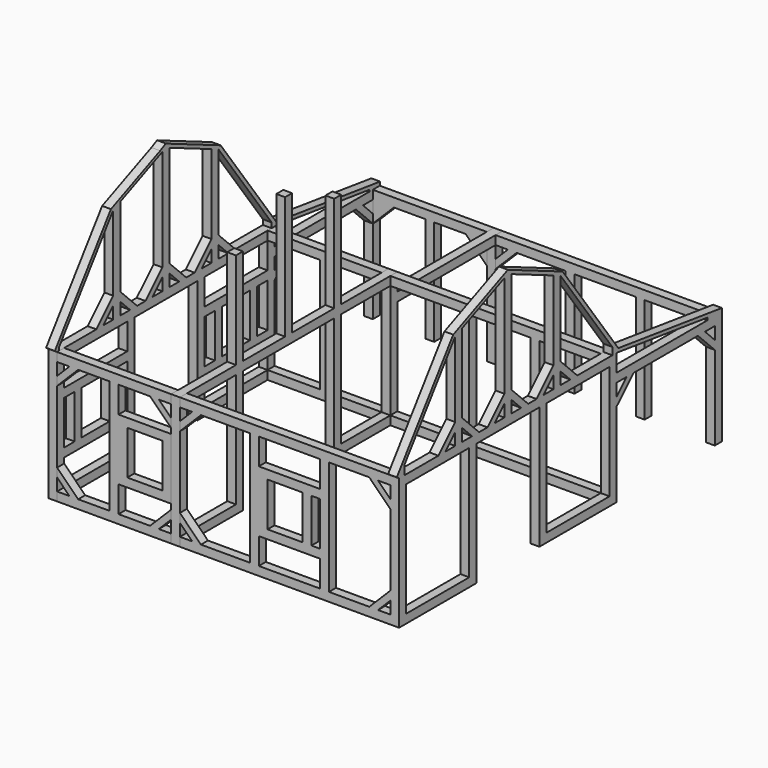
from build123d import *

# Parameters (mm, degrees)
F0_W      = 20
F0_H      = 25
F1_DEPTH  = 5
F0_W_2    = 35
F0_H_2    = 15
F0_W_3    = 5
F2_W      = 7.5
F2_H      = 25
F2_W_2    = 45
F2_H_2    = 15
F2_H_3    = 24.9999969228
F2_W_3    = 20
F3_DEPTH  = 5
F4_W      = 45
F4_H      = 65
F5_DEPTH  = 5
F6_W      = 35
F6_H      = 65
F7_DEPTH  = 5
F8_W      = 35
F8_H      = 65
F9_DEPTH  = 5
F11_DEPTH = 5


# Not quite as in the source:
# - ends of sketch curves that miss each other by under 0.0002 mm in the source are joined


with BuildPart() as f1:
    # F0 (on Front) → F1 (new body)
    with BuildSketch(Plane.XZ):
        Polygon((-8.9761292934, 70), (-73.9761292934, 70), (-73.9761292934, 65), (-66.9761292934, 65), (-73.9761292934, 58), (-73.9761292934, 53), (-61.9761292934, 65), (-43.9761292934, 65), (-43.9761292934, 0), (-61.9761292934, 0), (-73.9761292934, 12), (-73.9761292934, 7), (-66.9761292934, 0), (-73.9761292934, 0), (-73.9761292934, -5), (-8.9761292934, -5), (-8.9761292934, 0), (-15.9761292934, 0), (-8.9761292934, 7), (-8.9761292934, 12), (-20.9761292934, 0), (-38.9761292934, 0), (-38.9761292934, 15), (-8.9761292934, 15), (-8.9761292934, 50), (-38.9761292934, 50), (-38.9761292934, 65), (-20.9761292934, 65), (-8.9761292934, 53), (-8.9761292934, 58), (-15.9761292934, 65), (-8.9761292934, 65), align=None)
        with Locations((-23.9761292934, 32.5)):
            Rectangle(F0_W, F0_H, mode=Mode.SUBTRACT)
    extrude(amount=F1_DEPTH)


with BuildPart() as f1b:
    # F0 (on Front) → F1, piece 2 (new body)
    with BuildSketch(Plane.XZ):
        Polygon((-3.9761292934, -5), (116.0238707066, -5), (116.0238707066, 0), (109.0238707066, 0), (116.0238707066, 7), (116.0238707066, 12), (104.0238707066, 0), (81.0238707066, 0), (81.0238707066, 65), (104.0238707066, 65), (116.0238707066, 53), (116.0238707066, 58), (109.0238707066, 65), (116.0238707066, 65), (116.0238707066, 70), (-3.9761292934, 70), (-3.9761292934, 65), (3.0238707066, 65), (-3.9761292934, 58), (-3.9761292934, 53), (8.0238707066, 65), (36.0238707066, 65), (36.0238707066, 0), (8.0238707066, 0), (-3.9761292934, 12), (-3.9761292934, 7), (3.0238707066, 0), (-3.9761292934, 0), align=None)
        with Locations((58.5238707066, 7.5)):
            Rectangle(F0_W_2, F0_H_2, mode=Mode.SUBTRACT)
        with Locations((56.0238707066, 32.5)):
            Rectangle(F0_W, F0_H, mode=Mode.SUBTRACT)
        with Locations((73.5238707066, 32.5)):
            Rectangle(F0_W_3, F0_H, mode=Mode.SUBTRACT)
        with Locations((58.5238707066, 57.5)):
            Rectangle(F0_W_2, F0_H_2, mode=Mode.SUBTRACT)
    extrude(amount=F1_DEPTH)

    # F4 (on face) → F5 (join)
    with BuildSketch(Plane.YZ.offset(116.0238707066)):
        Polygon((-5, 70), (-5, -5), (50, -5), (50, 65), (95, 65), (95, -5), (150, -5), (150, 43), (162, 55), (208, 55), (220, 43), (220, -5), (225, -5), (225.0925493266, 62.0075330331), (151.2473517716, 71.8535593737), (111.5438002141, 126.4459427654), (72.5, 143.179), (33.5786001005, 126.4459427654), (-6.6174721686, 71.1763433954), align=None)
        with Locations((22.5, 32.5)):
            Rectangle(F4_W, F4_H, mode=Mode.SUBTRACT)
        with Locations((122.5, 32.5)):
            Rectangle(F4_W, F4_H, mode=Mode.SUBTRACT)
        Polygon((150, 48), (150, 55), (157, 55), align=None, mode=Mode.SUBTRACT)
        Polygon((214.6482616663, 60), (150, 60), (150, 70), (214.6482616663, 61.3802317778), align=None, mode=Mode.SUBTRACT)
        Polygon((213, 55), (220, 55), (220, 48), align=None, mode=Mode.SUBTRACT)
        Polygon((35, 77), (35, 70), (28, 70), align=None, mode=Mode.SUBTRACT)
        Polygon((47, 70), (40, 70), (40, 77), align=None, mode=Mode.SUBTRACT)
        Polygon((35, 82), (23, 70), (-0.9940898744, 70), (-0.9940898744, 75.5081264226), (35, 125), align=None, mode=Mode.SUBTRACT)
        Polygon((70, 77), (70, 70), (63, 70), align=None, mode=Mode.SUBTRACT)
        Polygon((82, 70), (75, 70), (75, 77), align=None, mode=Mode.SUBTRACT)
        Polygon((105, 77), (105, 70), (98, 70), align=None, mode=Mode.SUBTRACT)
        Polygon((70, 82), (58, 70), (52, 70), (40, 82), (40, 127.1428571429), (70, 140), align=None, mode=Mode.SUBTRACT)
        Polygon((105, 82), (93, 70), (87, 70), (75, 82), (75, 140), (105, 127.1428571429), align=None, mode=Mode.SUBTRACT)
        Polygon((117, 70), (110, 70), (110, 77), align=None, mode=Mode.SUBTRACT)
        Polygon((146.9582170248, 70), (122, 70), (110, 82), (110, 125), (146.9582170248, 74.1824515909), align=None, mode=Mode.SUBTRACT)
    extrude(amount=F5_DEPTH)


with BuildPart() as f3:
    # F2 (on face) → F3 (new body)
    with BuildSketch(Plane(origin=(-73.9761292934, 0, 0), x_dir=(0, -1, 0), z_dir=(-1, 0, 0))):
        Polygon((-50, -5), (5, -5), (5, 70), (6.6174721686, 71.1763433954), (-33.3458997011, 126.1259797162), (-68.4692735837, 141.1788542373), (-72.4999997374, 143.1788542373), (-76.1898970514, 141.5453457622), (-111.5439879277, 126.3935925295), (-151.2089944152, 71.8542086093), (-225.2643269151, 61.9801642759), (-224.9999994749, 59.9977084746), (-224.9999994749, -5.0022915254), (-219.9999994749, -5.0022915254), (-219.9999994749, 43), (-208, 54.9977084746), (-162, 54.9977084746), (-149.9993812049, 43.0000000159), (-149.996908125, -4.9999999204), (-94.996908198, -4.997166183), (-95.0005147729, 65.0028337241), (-50, 65), align=None)
        Polygon((-99.9999995346, 0.0023185124), (-144.9999994749, 0), (-144.9999994749, 15), (-99.9999995208, 15.0023185124), align=None, mode=Mode.SUBTRACT)
        Polygon((-219.9999994749, 48), (-219.9999994749, 54.9977084746), (-213, 54.9977084746), align=None, mode=Mode.SUBTRACT)
        Polygon((-217.5258704674, 60.9942590089), (-149.9999994749, 69.9977084746), (-149.9999994749, 59.9977084746), (-217.5258704674, 59.9977084746), align=None, mode=Mode.SUBTRACT)
        with Locations((-141.2499994749, 32.5)):
            Rectangle(F2_W, F2_H, mode=Mode.SUBTRACT)
        Polygon((-112.4999995096, 20.0020609068), (-132.4999994749, 20), (-132.4999994749, 45), (-112.4999995162, 45.0023185193), align=None, mode=Mode.SUBTRACT)
        Polygon((-157, 54.9977084746), (-149.9999994749, 54.9977084746), (-149.9996388174, 48.0000000093), align=None, mode=Mode.SUBTRACT)
        Polygon((-144.9999994749, 50), (-144.9999994749, 65), (-99.9999994749, 65), (-99.9999994887, 50.0023154352), align=None, mode=Mode.SUBTRACT)
        with Locations((-22.5, 7.5)):
            Rectangle(F2_W_2, F2_H_2, mode=Mode.SUBTRACT)
        with Locations((-103.7499995162, 32.5023169738)):
            Rectangle(F2_W, F2_H_3, mode=Mode.SUBTRACT)
        with Locations((-41.25, 32.5)):
            Rectangle(F2_W, F2_H, mode=Mode.SUBTRACT)
        with Locations((-22.5, 32.5)):
            Rectangle(F2_W_3, F2_H, mode=Mode.SUBTRACT)
        with Locations((-3.75, 32.5)):
            Rectangle(F2_W, F2_H, mode=Mode.SUBTRACT)
        with Locations((-22.5, 57.5)):
            Rectangle(F2_W_2, F2_H_2, mode=Mode.SUBTRACT)
        Polygon((-109.9999994749, 76.9977084746), (-109.9999994749, 69.9977084746), (-116.9999994749, 69.9977084746), align=None, mode=Mode.SUBTRACT)
        Polygon((-109.9999994749, 81.9977084746), (-121.9999994749, 69.9977084746), (-147.8956698396, 69.9977084746), (-147.8956698396, 72.8911617231), (-109.9999994749, 124.9977084746), align=None, mode=Mode.SUBTRACT)
        Polygon((-97.9999994749, 69.9977084746), (-104.9999994749, 69.9977084746), (-104.9999994749, 76.9977084746), align=None, mode=Mode.SUBTRACT)
        Polygon((-74.9999994749, 76.9977084746), (-74.9999994749, 69.9977084746), (-81.9999994749, 69.9977084746), align=None, mode=Mode.SUBTRACT)
        Polygon((-63, 70), (-70, 70), (-70, 76.9977084746), align=None, mode=Mode.SUBTRACT)
        Polygon((-86.9999994749, 69.9977084746), (-92.9999994749, 69.9977084746), (-104.9999994749, 81.9977084746), (-104.9999994749, 127.1405656174), (-74.9999994749, 139.9977084746), (-74.9999994749, 81.9977084746), align=None, mode=Mode.SUBTRACT)
        Polygon((-52, 70), (-58, 70), (-70, 81.9977084746), (-70, 140), (-40, 127.1428571429), (-40, 81.9977084746), align=None, mode=Mode.SUBTRACT)
        Polygon((-40, 76.9977084746), (-40, 70), (-47, 70), align=None, mode=Mode.SUBTRACT)
        Polygon((-28, 70), (-35, 70), (-35, 76.9977084746), align=None, mode=Mode.SUBTRACT)
        Polygon((3.6190291482, 70), (-23, 70), (-35, 81.9977084746), (-35, 125), (3.6190291482, 71.8988349212), align=None, mode=Mode.SUBTRACT)
    extrude(amount=F3_DEPTH)


with BuildPart() as f7:
    # F6 (on face) → F7 (new body)
    with BuildSketch(Plane(origin=(0, 150, 0), x_dir=(-1, 0, 0), z_dir=(0, 1, 0))):
        Polygon((3.9761292934, 0), (-36.0238707066, 0), (-36.0238707066, 65), (3.9761292934, 65), (3.9761292934, 70), (-116.0238707066, 70), (-116.0238707066, 65), (-81.0238707066, 65), (-81.0238707066, 0), (-116.0238707066, 0), (-116.0238707066, -5), (3.9761292934, -5), align=None)
        with Locations((-58.5238707066, 32.5)):
            Rectangle(F6_W, F6_H, mode=Mode.SUBTRACT)
    extrude(amount=-F7_DEPTH)


with BuildPart() as f7b:
    # F6 (on face) → F7, piece 2 (new body)
    with BuildSketch(Plane(origin=(0, 150, 0), x_dir=(-1, 0, 0), z_dir=(0, 1, 0))):
        Polygon((73.9761292934, 70), (8.9761292934, 70), (8.9761292934, 65), (38.9761292934, 65), (38.9761292934, 0), (8.9761292934, 0), (8.9761292934, -5), (73.9761292934, -5), (73.9761292934, 0), (43.9761292934, 0), (43.9761292934, 65), (73.9761292934, 65), align=None)
    extrude(amount=-F7_DEPTH)


with BuildPart() as f9:
    # F8 (on face) → F9 (new body)
    with BuildSketch(Plane.YZ.offset(-8.9761292934)):
        Polygon((35, 70), (-5, 70), (-5, -5), (40, -5), (40, 65), (105, 65), (105, -5), (150, -5), (150, 55), (150, 60), (150, 70), (110, 70), (110, 125), (105, 125), (105, 70), (75, 70), (75, 140), (70, 140), (70, 70), (40, 70), (40, 125), (35, 125), align=None)
        with Locations((17.5, 32.5)):
            Rectangle(F8_W, F8_H, mode=Mode.SUBTRACT)
        with Locations((127.5, 32.5)):
            Rectangle(F8_W, F8_H, mode=Mode.SUBTRACT)
        Polygon((150, 60), (150, 55), (220, 55), (220, -5), (225, -5), (225, 60), align=None)
    extrude(amount=F9_DEPTH)


with BuildPart() as f11:
    # F10 (on face) → F11 (new body)
    with BuildSketch(Plane(origin=(0, 224.9999994749, 0), x_dir=(-1, 0, 0), z_dir=(0, 1, 0))):
        Polygon((-116.0238707066, 48), (-116.0238707066, 43), (-104.0238707066, 55), (-81.0238707066, 55), (-81.0238707066, -5), (-76.0238707066, -5), (-76.0238707066, 55), (-41.0238707066, 55), (-41.0238707066, -5), (-36.0238707066, -5), (-36.0238707066, 55), (-8.0238707066, 55), (3.9761292934, 43), (3.9761292934, 48), (-3.0238707066, 55), (3.9761292934, 55), (3.9761292934, 60), (-116.0238707066, 60), (-116.0238707066, 55), (-109.0238707066, 55), align=None)
    extrude(amount=-F11_DEPTH)


with BuildPart() as f11b:
    # F10 (on face) → F11, piece 2 (new body)
    with BuildSketch(Plane(origin=(0, 224.9999994749, 0), x_dir=(-1, 0, 0), z_dir=(0, 1, 0))):
        Polygon((73.9761292934, 59.9977084746), (8.9761292934, 59.9977084746), (8.9761292934, 54.9977084746), (15.9761292934, 54.9977084746), (20.9761292934, 54.9977084746), (38.9761292934, 54.9977084746), (38.9761292934, -5.0022915254), (43.9761292934, -5.0022915254), (43.9761292934, 54.9977084746), (61.9761292934, 54.9977084746), (66.9761292934, 54.9977084746), (73.9761292934, 54.9977084746), align=None)
        Polygon((15.9761292934, 54.9977084746), (8.9761292934, 54.9977084746), (8.9761292934, 47.9977084746), align=None)
        Polygon((73.9761292934, 47.9977084746), (73.9761292934, 54.9977084746), (66.9761292934, 54.9977084746), align=None)
        Polygon((20.9761292934, 54.9977084746), (15.9761292934, 54.9977084746), (8.9761292934, 47.9977084746), (8.9761292934, 42.9977084746), align=None)
        Polygon((73.9761292934, 47.9977084746), (66.9761292934, 54.9977084746), (61.9761292934, 54.9977084746), (73.9761292934, 42.9977084746), align=None)
    extrude(amount=-F11_DEPTH)


solid = Compound([f1.part, f1b.part, f3.part, f7.part, f7b.part, f9.part, f11.part, f11b.part])
